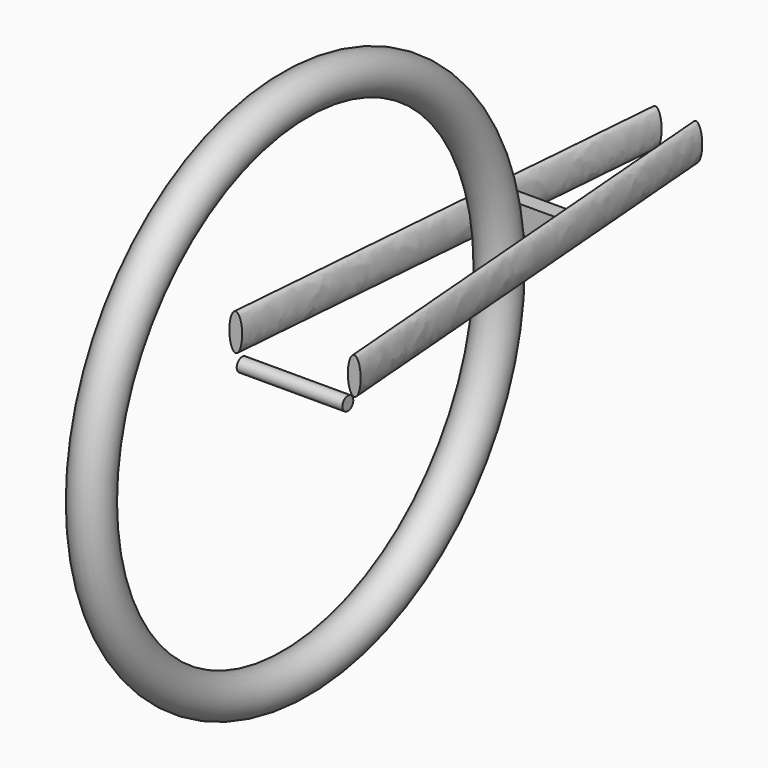
from build123d import *

# Parameters (mm, degrees)
F4_R     = 8.5
F5_DEPTH = 132
F8_R     = 25
F16_W    = 20.2121138573
F16_H    = 33.3737321198


# Not quite as in the source:
# - the program builds the solid bodies; features that only make, move or delete a surface that nothing else refers to are left out


with BuildPart() as f5:
    # F4 (on offset) → F5 (new body)
    with BuildSketch(Plane.YZ.offset(26)):
        Circle(F4_R)
    extrude(amount=F5_DEPTH)


with BuildPart() as f9:
    # F9: sweep along a path in F7
    with BuildLine(Plane.YZ.offset(92)) as f9_path:
        CenterArc((0, 0), 318, 0, 360)
    # F8 (on Front) → F9 (sweep)
    with BuildSketch(Plane.XZ):
        with Locations((92.3355445266, 318.2308673859)):
            Circle(F8_R)
    sweep(path=f9_path.line)


with BuildPart() as f12:
    # F12: sweep along a path in F10
    with BuildLine(Plane.XY.offset(32.8)) as f12_path:
        Line((166.0082890247, 0), (117.3492670059, 594.0103530884))
    # F11 (on Front) → F12 (sweep)
    with BuildSketch(Plane.XZ):
        with BuildLine():
            add(Edge.make_bspline(
                [(166.0082890247, 9.8), (179.8646954852, 9.8), (172.9364922549, 44.3), (166.0082890247, 78.8), (159.0800857944, 44.3), (152.1518825641, 9.8), (166.0082890247, 9.8)],
                knots=[0, 0, 0, 2.0943951024, 2.0943951024, 4.1887902048, 4.1887902048, 6.2831853072, 6.2831853072, 6.2831853072], degree=2, weights=[1, 0.5, 1, 0.5, 1, 0.5, 1]))
        make_face()
    sweep(path=f12_path.line)


with BuildPart() as f13_1:
    # F13: instance of F12
    add(f12.part.mirror(Plane.YZ.offset(92)))


with BuildPart() as f17:
    # F17: sweep along a path in F14
    with BuildLine(Plane.XY.offset(32.8)) as f17_path:
        Line((48.0404309928, 369.5430159569), (135.303452611, 369.5430159569))
    # F16 (on face) → F17 (sweep)
    with BuildSketch(Plane(origin=(164.9017569532, 13.5081117371, 0), x_dir=(-0.0816426544, 0.9966616663, 0), z_dir=(0.9966616663, 0.0816426544, 0))):
        with Locations((357.2628250169, 32.8)):
            Rectangle(F16_W, F16_H)
    sweep(path=f17_path.line)


solid = Compound([f5.part, f9.part, f12.part, f13_1.part, f17.part])
